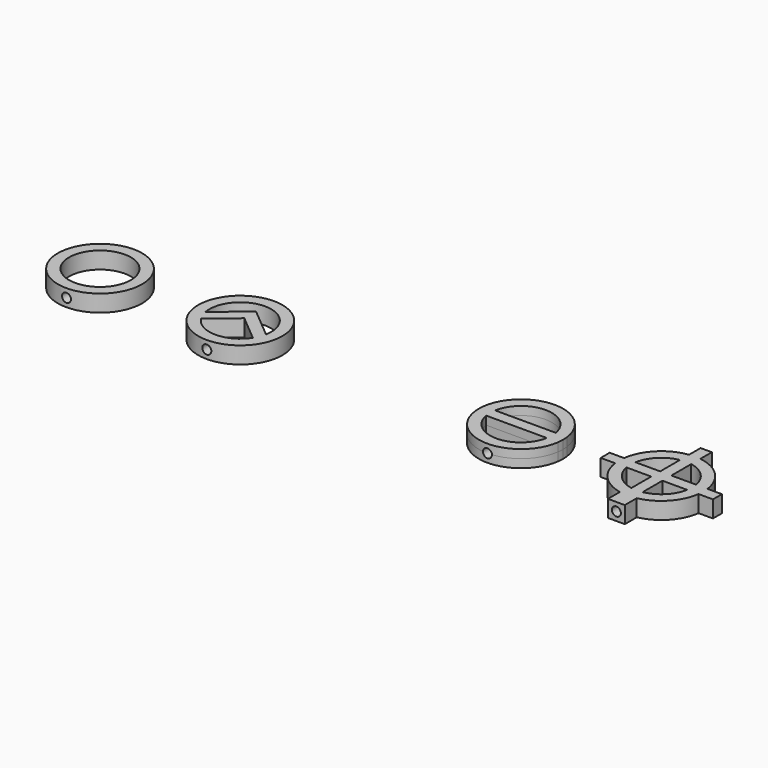
from build123d import *

# Parameters (mm, degrees)
F0_W     = 2
F0_H     = 2
F1_DEPTH = 1.5
F0_R     = 7.5
F0_R_2   = 5.5
F2_R     = 0.8
F3_DEPTH = 5


with BuildPart() as f1:
    # F0 (on Top) → F1 (new body, symmetric)
    with BuildSketch(Plane.XY):
        with BuildLine():
            ThreePointArc((57.4330343737, -1), (57.4832398666, -0.5011198447), (57.5, 0))
            ThreePointArc((57.5, 0), (57.4832398666, 0.5011198447), (57.4330343737, 1))
            Line((57.4330343737, 1), (55.4083269132, 1))
            ThreePointArc((55.4083269132, 1), (55.4770337785, 0.502096593), (55.5, 0))
            ThreePointArc((55.5, 0), (55.4770337785, -0.502096593), (55.4083269132, -1))
            Line((55.4083269132, -1), (57.4330343737, -1))
        make_face()
        with BuildLine():
            ThreePointArc((57.4330343737, 1), (57.4832398666, 0.5011198447), (57.5, 0))
            ThreePointArc((57.5, 0), (57.4832398666, -0.5011198447), (57.4330343737, -1))
            Line((57.4330343737, -1), (60, -1))
            Line((60, -1), (60, 1))
            Line((60, 1), (57.4330343737, 1))
        make_face()
        with BuildLine():
            Line((55.4083269132, 1), (57.4330343737, 1))
            ThreePointArc((57.4330343737, 1), (55.3033008589, 5.3033008589), (51, 7.4330343737))
            Line((51, 7.4330343737), (51, 5.4083269132))
            ThreePointArc((51, 5.4083269132), (53.8890872965, 3.8890872965), (55.4083269132, 1))
        make_face()
        with BuildLine():
            ThreePointArc((51.5, -7.3484692283), (55.4795566578, -5.1209822138), (57.4330343737, -1))
            Line((57.4330343737, -1), (55.4083269132, -1))
            ThreePointArc((55.4083269132, -1), (53.8890872965, -3.8890872965), (51, -5.4083269132))
            Line((51, -5.4083269132), (51, -7.3484692283))
            Line((51, -7.3484692283), (51.5, -7.3484692283))
        make_face()
        with BuildLine():
            Line((51, 5.4083269132), (51, 7.4330343737))
            ThreePointArc((51, 7.4330343737), (50, 7.5), (49, 7.4330343737))
            Line((49, 7.4330343737), (49, 5.4083269132))
            ThreePointArc((49, 5.4083269132), (50, 5.5), (51, 5.4083269132))
        make_face()
        with BuildLine():
            ThreePointArc((49, 7.4330343737), (50, 7.5), (51, 7.4330343737))
            Line((51, 7.4330343737), (51, 10))
            Line((51, 10), (49, 10))
            Line((49, 10), (49, 7.4330343737))
        make_face()
        with BuildLine():
            ThreePointArc((55.5, 0), (55.4770337785, 0.502096593), (55.4083269132, 1))
            Line((55.4083269132, 1), (51, 1))
            Line((51, 1), (51, -1))
            Line((51, -1), (55.4083269132, -1))
            ThreePointArc((55.4083269132, -1), (55.4770337785, -0.502096593), (55.5, 0))
        make_face()
        with BuildLine():
            Line((51.5, -10), (51.5, -7.3484692283))
            ThreePointArc((51.5, -7.3484692283), (51.2507149219, -7.3949788495), (51, -7.4330343737))
            Line((51, -7.4330343737), (51, -10))
            Line((51, -10), (51.5, -10))
        make_face()
        with BuildLine():
            ThreePointArc((51, -7.4330343737), (51.2507149219, -7.3949788495), (51.5, -7.3484692283))
            Line((51.5, -7.3484692283), (51, -7.3484692283))
            Line((51, -7.3484692283), (51, -7.4330343737))
        make_face()
        with BuildLine():
            Line((49, 5.4083269132), (49, 7.4330343737))
            ThreePointArc((49, 7.4330343737), (44.6966991411, 5.3033008589), (42.5669656263, 1))
            Line((42.5669656263, 1), (44.5916730868, 1))
            ThreePointArc((44.5916730868, 1), (46.1109127035, 3.8890872965), (49, 5.4083269132))
        make_face()
        with BuildLine():
            Line((51, 1), (51, 5.4083269132))
            ThreePointArc((51, 5.4083269132), (50, 5.5), (49, 5.4083269132))
            Line((49, 5.4083269132), (49, 1))
            Line((49, 1), (51, 1))
        make_face()
        with Locations((50, 0)):
            Rectangle(F0_W, F0_H)
        with BuildLine():
            Line((51, -10), (51, -7.4330343737))
            ThreePointArc((51, -7.4330343737), (50, -7.5), (49, -7.4330343737))
            Line((49, -7.4330343737), (49, -10))
            Line((49, -10), (51, -10))
        make_face()
        with BuildLine():
            ThreePointArc((49, -7.4330343737), (50, -7.5), (51, -7.4330343737))
            Line((51, -7.4330343737), (51, -7.3484692283))
            Line((51, -7.3484692283), (49, -7.3484692283))
            Line((49, -7.3484692283), (49, -7.4330343737))
        make_face()
        with BuildLine():
            Line((49, -7.3484692283), (51, -7.3484692283))
            Line((51, -7.3484692283), (51, -5.4083269132))
            ThreePointArc((51, -5.4083269132), (50, -5.5), (49, -5.4083269132))
            Line((49, -5.4083269132), (49, -7.3484692283))
        make_face()
        with BuildLine():
            ThreePointArc((49, -5.4083269132), (50, -5.5), (51, -5.4083269132))
            Line((51, -5.4083269132), (51, -1))
            Line((51, -1), (49, -1))
            Line((49, -1), (49, -5.4083269132))
        make_face()
        with BuildLine():
            Line((44.5916730868, 1), (42.5669656263, 1))
            ThreePointArc((42.5669656263, 1), (42.5, 0), (42.5669656263, -1))
            Line((42.5669656263, -1), (44.5916730868, -1))
            ThreePointArc((44.5916730868, -1), (44.5, 0), (44.5916730868, 1))
        make_face()
        with BuildLine():
            ThreePointArc((42.5669656263, -1), (42.5, 0), (42.5669656263, 1))
            Line((42.5669656263, 1), (40, 1))
            Line((40, 1), (40, -1))
            Line((40, -1), (42.5669656263, -1))
        make_face()
        with BuildLine():
            Line((49, -1), (49, 1))
            Line((49, 1), (44.5916730868, 1))
            ThreePointArc((44.5916730868, 1), (44.5, 0), (44.5916730868, -1))
            Line((44.5916730868, -1), (49, -1))
        make_face()
        with BuildLine():
            Line((49, -10), (49, -7.4330343737))
            ThreePointArc((49, -7.4330343737), (48.7492850781, -7.3949788495), (48.5, -7.3484692283))
            Line((48.5, -7.3484692283), (48.5, -10))
            Line((48.5, -10), (49, -10))
        make_face()
        with BuildLine():
            ThreePointArc((48.5, -7.3484692283), (48.7492850781, -7.3949788495), (49, -7.4330343737))
            Line((49, -7.4330343737), (49, -7.3484692283))
            Line((49, -7.3484692283), (48.5, -7.3484692283))
        make_face()
        with BuildLine():
            Line((48.5, -7.3484692283), (49, -7.3484692283))
            Line((49, -7.3484692283), (49, -5.4083269132))
            ThreePointArc((49, -5.4083269132), (46.1109127035, -3.8890872965), (44.5916730868, -1))
            Line((44.5916730868, -1), (42.5669656263, -1))
            ThreePointArc((42.5669656263, -1), (44.5204433422, -5.1209822138), (48.5, -7.3484692283))
        make_face()
    extrude(amount=F1_DEPTH, both=True)


with BuildPart() as f1b:
    # F0 (on Top) → F1, piece 2 (new body, symmetric)
    with BuildSketch(Plane.XY):
        with BuildLine():
            ThreePointArc((32.4330343737, -1), (32.4832398666, -0.5011198447), (32.5, 0))
            ThreePointArc((32.5, 0), (32.4832398666, 0.5011198447), (32.4330343737, 1))
            Line((32.4330343737, 1), (32.4330343737, -1))
        make_face()
        with BuildLine():
            Line((30.4083269132, 1), (32.4330343737, 1))
            ThreePointArc((32.4330343737, 1), (25, 7.5), (17.5669656263, 1))
            Line((17.5669656263, 1), (19.5916730868, 1))
            ThreePointArc((19.5916730868, 1), (25, 5.5), (30.4083269132, 1))
        make_face()
        with BuildLine():
            Line((32.4330343737, -1), (32.4330343737, 1))
            Line((32.4330343737, 1), (30.4083269132, 1))
            ThreePointArc((30.4083269132, 1), (30.4770337785, 0.502096593), (30.5, 0))
            ThreePointArc((30.5, 0), (30.4770337785, -0.502096593), (30.4083269132, -1))
            Line((30.4083269132, -1), (32.4330343737, -1))
        make_face()
        with BuildLine():
            ThreePointArc((17.5669656263, -1), (25, -7.5), (32.4330343737, -1))
            Line((32.4330343737, -1), (30.4083269132, -1))
            ThreePointArc((30.4083269132, -1), (25, -5.5), (19.5916730868, -1))
            Line((19.5916730868, -1), (17.5669656263, -1))
        make_face()
        with BuildLine():
            Line((17.5669656263, -1), (17.5669656263, 1))
            ThreePointArc((17.5669656263, 1), (17.5, 0), (17.5669656263, -1))
        make_face()
        with BuildLine():
            Line((19.5916730868, 1), (17.5669656263, 1))
            Line((17.5669656263, 1), (17.5669656263, -1))
            Line((17.5669656263, -1), (19.5916730868, -1))
            ThreePointArc((19.5916730868, -1), (19.5, 0), (19.5916730868, 1))
        make_face()
        with BuildLine():
            ThreePointArc((30.5, 0), (30.4770337785, 0.502096593), (30.4083269132, 1))
            Line((30.4083269132, 1), (19.5916730868, 1))
            ThreePointArc((19.5916730868, 1), (19.5, 0), (19.5916730868, -1))
            Line((19.5916730868, -1), (30.4083269132, -1))
            ThreePointArc((30.4083269132, -1), (30.4770337785, -0.502096593), (30.5, 0))
        make_face()
    extrude(amount=F1_DEPTH, both=True)


with BuildPart() as f1c:
    # F0 (on Top) → F1, piece 3 (new body, symmetric)
    with BuildSketch(Plane.XY):
        with Locations((-25, 0)):
            Circle(F0_R)
        with BuildLine():
            ThreePointArc((-30.4021345309, -1.0329290925), (-25.5187774475, 5.4754789708), (-19.5, 0))
            ThreePointArc((-19.5, 0), (-19.5245210292, -0.5187774475), (-19.5978654691, -1.0329290925))
            ThreePointArc((-19.5978654691, -1.0329290925), (-19.8953014496, -2.0474502947), (-20.38135333, -2.986319296))
            ThreePointArc((-20.38135333, -2.986319296), (-25, -5.5), (-29.61864667, -2.986319296))
            ThreePointArc((-29.61864667, -2.986319296), (-30.1046985504, -2.0474502947), (-30.4021345309, -1.0329290925))
        make_face(mode=Mode.SUBTRACT)
        with BuildLine():
            Line((-25, 3.5), (-30.4021345309, -1.0329290925))
            ThreePointArc((-30.4021345309, -1.0329290925), (-30.1046985504, -2.0474502947), (-29.61864667, -2.986319296))
            Line((-29.61864667, -2.986319296), (-25, 0.8891854213))
            Line((-25, 0.8891854213), (-20.38135333, -2.986319296))
            ThreePointArc((-20.38135333, -2.986319296), (-19.8953014496, -2.0474502947), (-19.5978654691, -1.0329290925))
            Line((-19.5978654691, -1.0329290925), (-25, 3.5))
        make_face()
    extrude(amount=F1_DEPTH, both=True)


with BuildPart() as f1d:
    # F0 (on Top) → F1, piece 4 (new body, symmetric)
    with BuildSketch(Plane.XY):
        with Locations((-50, 0)):
            Circle(F0_R)
        with Locations((-50, 0)):
            Circle(F0_R_2, mode=Mode.SUBTRACT)
    extrude(amount=F1_DEPTH, both=True)


with BuildPart() as f3_tool:
    # F2 (on face) → F3 (new body)
    with BuildSketch(Plane.XZ.offset(10)):
        with Locations((50, 0)):
            Circle(F2_R)
        with Locations((25, 0)):
            Circle(F2_R)
        with Locations((-25, 0)):
            Circle(F2_R)
        with Locations((-50, 0)):
            Circle(F2_R)
    extrude(amount=-F3_DEPTH)


with BuildPart() as f1_1:
    add(f1.part)

    # F3: cut by f3_tool
    add(f3_tool.part, mode=Mode.SUBTRACT)


with BuildPart() as f1b_1:
    add(f1b.part)

    # F3: cut by f3_tool
    add(f3_tool.part, mode=Mode.SUBTRACT)


with BuildPart() as f1c_1:
    add(f1c.part)

    # F3: cut by f3_tool
    add(f3_tool.part, mode=Mode.SUBTRACT)


with BuildPart() as f1d_1:
    add(f1d.part)

    # F3: cut by f3_tool
    add(f3_tool.part, mode=Mode.SUBTRACT)


solid = Compound([f1_1.part, f1b_1.part, f1c_1.part, f1d_1.part])
